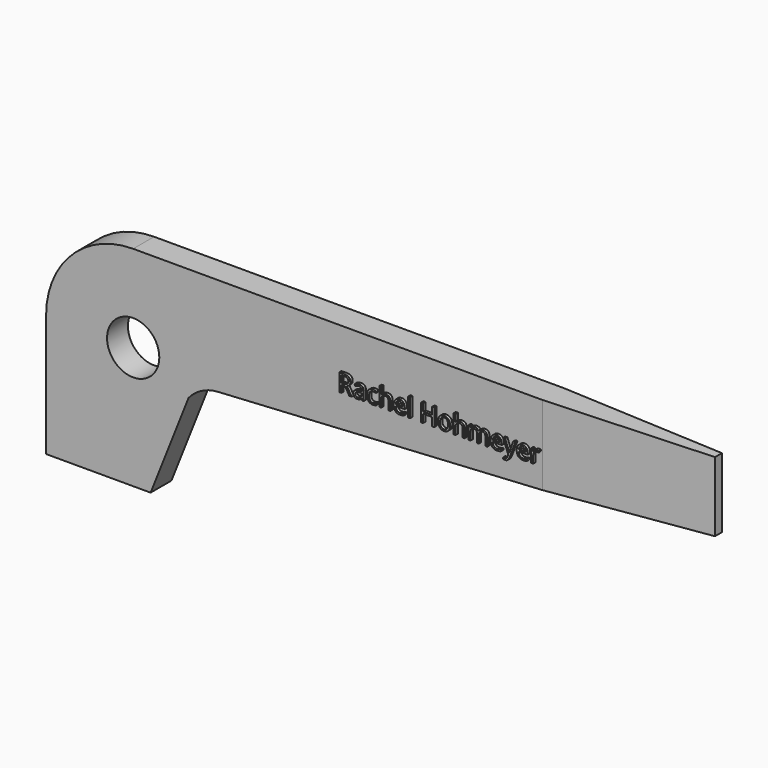
from build123d import *

# Parameters (mm, degrees)
F1_DEPTH     = 2.38125
F2_R         = 2.38125
F3_DEPTH     = 2.38225
F5_DEPTH     = 25.4
F6_TEXT_SIZE = 2.23082583
F7_DEPTH     = 0.254


# Not quite as in the source:
# - Text() gives the source's letters only with a copy of the font that has no kerning and outlines rounded to 1/6400 em; it was checked with that copy


with BuildPart() as f1:
    # F0 (on Front) → F1 (new body)
    with BuildSketch(Plane.XZ):
        with BuildLine():
            Line((60.325, 19.05), (7.9375, 19.05))
            ThreePointArc((7.9375, 19.05), (2.3248399243, 16.7251600757), (0, 11.1125))
            Line((0, 11.1125), (0, 0))
            Line((0, 0), (9.525, 0))
            Line((9.525, 0), (12.9771089609, 8.7189015115))
            ThreePointArc((12.9771089609, 8.7189015115), (14.1733071246, 9.6837228744), (15.6563832798, 10.0865322928))
            Line((15.6563832798, 10.0865322928), (60.325, 12.7))
            Line((60.325, 12.7), (60.325, 19.05))
        make_face()
    extrude(amount=F1_DEPTH)

    # F2 (on face) → F3 (cut, through all)
    with BuildSketch(Plane.XZ.offset(2.38125)):
        with Locations((7.9375, 11.1125)):
            Circle(F2_R)
    extrude(amount=-F3_DEPTH, mode=Mode.SUBTRACT)

    # F4 (on face) → F5 (cut)
    with BuildSketch(Plane.XY.offset(19.05)):
        Polygon((60.325, 0), (45.24375, 0), (60.325, -0.79375), align=None)
        Polygon((60.325, -2.38125), (60.325, -1.5875), (45.24375, -2.38125), align=None)
    extrude(amount=-F5_DEPTH, mode=Mode.SUBTRACT)

    # F6 (on face) → F7 (join)
    with BuildSketch(Plane.XZ.offset(2.38125)):
        with Locations((26.7083758846, 13.8276191428)):
            Text('Rachel Hohmeyer', F6_TEXT_SIZE, font='Open Sans', text_align=(TextAlign.LEFT, TextAlign.BOTTOM))
    extrude(amount=F7_DEPTH)


solid = f1.part
